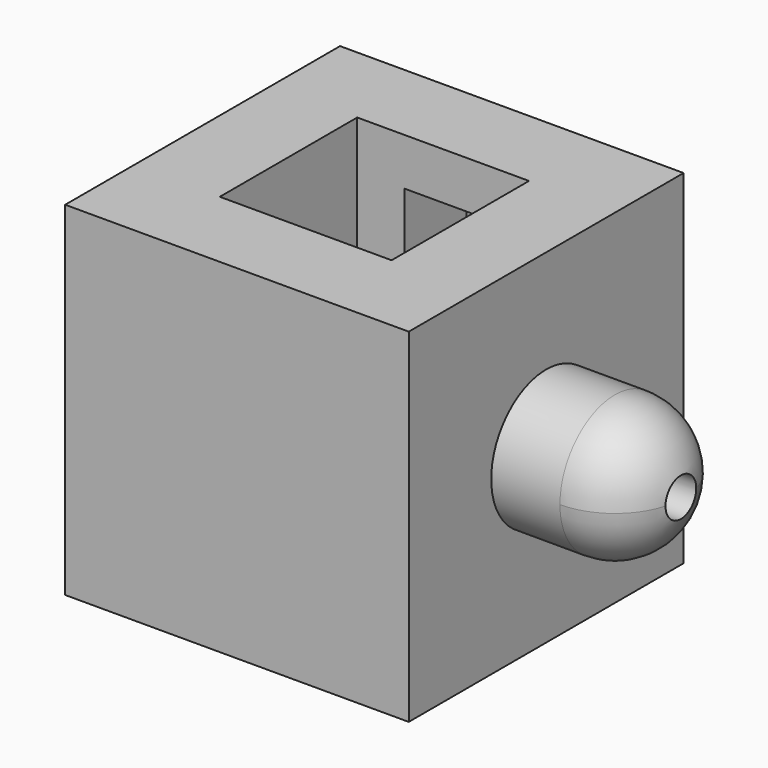
from build123d import *

# Parameters (mm, degrees)
F0_W           = 5
F0_H           = 5
F2_DEPTH       = 5
F3_W           = 2.5
F3_H           = 2.5
F4_DEPTH       = 2.5
F5_W           = 1.125
F5_H           = 1.125
F6_DEPTH       = 1.125
F7_R           = 1
F8_DEPTH       = 1
F10_ANGLE      = 180
F11_R          = 0.2796205341
F12_DEPTH      = 25.4
F13_DEPTH      = 2
F13_DEPTH_BACK = 5


# Not quite as in the source:
# - the program builds the solid bodies; features that only make, move or delete a surface that nothing else refers to are left out


with BuildPart() as f2:
    # F0 (on Top) → F2 (new body)
    with BuildSketch(Plane.XY):
        with Locations((2.5, -2.5)):
            Rectangle(F0_W, F0_H)
    extrude(amount=F2_DEPTH)

    # F3 (on face) → F4 (cut)
    with BuildSketch(Plane.XY.offset(5)):
        with Locations((2.5, -2.5)):
            Rectangle(F3_W, F3_H)
    extrude(amount=-F4_DEPTH, mode=Mode.SUBTRACT)

    # F5 (on face) → F6 (cut)
    with BuildSketch(Plane.XZ.offset(1.25)):
        with Locations((2.5, 3.75)):
            Rectangle(F5_W, F5_H)
    extrude(amount=-F6_DEPTH, mode=Mode.SUBTRACT)

    # F7 (on face) → F8 (join)
    with BuildSketch(Plane.YZ.offset(5)):
        with Locations((-2.5, 2.5)):
            Circle(F7_R)
    extrude(amount=F8_DEPTH)

    # F9 (on face) → F10 (revolve)
    with BuildSketch(Plane.YZ.offset(6)):
        with BuildLine():
            ThreePointArc((-1.5, 2.5), (-1.7928932188, 3.2071067812), (-2.5, 3.5))
            Line((-2.5, 3.5), (-2.5, 1.5))
            ThreePointArc((-2.5, 1.5), (-1.7928932188, 1.7928932188), (-1.5, 2.5))
        make_face()
    revolve(axis=Axis((6, -2.5, 2.5), (0, 0, -1)), revolution_arc=F10_ANGLE)

    # F11 (on face) → F12 (cut)
    with BuildSketch(Plane.YZ.offset(5)):
        with Locations((-2.5, 2.5)):
            Circle(F11_R)
    extrude(amount=F12_DEPTH, mode=Mode.SUBTRACT)

    # F11 (on face) → F13 (cut, two sides)
    with BuildSketch(Plane.YZ.offset(5)) as f13_sk:
        with Locations((-2.5, 2.5)):
            Circle(F11_R)
    extrude(amount=F13_DEPTH, mode=Mode.SUBTRACT)
    extrude(f13_sk.sketch, amount=-F13_DEPTH_BACK, mode=Mode.SUBTRACT)


solid = f2.part
